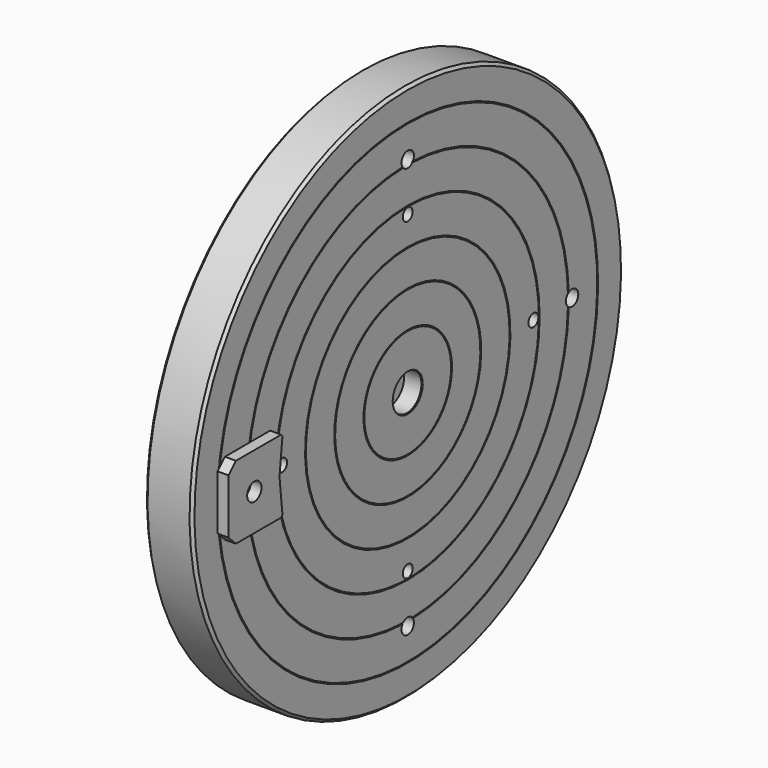
from build123d import *

# Parameters (mm, degrees)
F3_D            = 8.5
F3_DEPTH        = 20
F3_TIP          = 2.5536576309
F6_SIZE         = 1.5
F8_D            = 6.8
F10_D           = 8.5
F10_CBORE_D     = 20
F10_CBORE_DEPTH = 10
F12_D           = 8.5
F12_DEPTH       = 20
F12_TIP         = 2.5536576309
F13_R           = 4.9
F14_DEPTH       = 6
F15_SIZE        = 5
F16_SIZE        = 1


with BuildPart() as f1:
    # F0 (on Front) → F1 (revolve)
    with BuildSketch(Plane.XZ):
        Polygon((0, 80), (0, 62.5), (4, 62.5), (4, 0), (28, 0), (28, 147.5), (2, 147.5), (2, 80), align=None)
    revolve(axis=Axis((16, 0, 0), (1, 0, 0)))

    # F3
    with Locations(Plane(origin=(0, 0, 0), x_dir=(0, -1, 0), z_dir=(-1, 0, 0))):
        with Locations((0, 70), (60.6217782649, 35), (60.6217782649, -35), (0, -70), (-60.6217782649, -35), (-60.6217782649, 35)):
            Hole(F3_D / 2, depth=F3_DEPTH)
            with Locations((0, 0, -(F3_DEPTH + F3_TIP / 2))):  # 118° drill point
                Cone(0, F3_D / 2, F3_TIP, mode=Mode.SUBTRACT)

    # F4 (on Front) → F5 (revolve, cut)
    with BuildSketch(Plane.XZ):
        Polygon((28, 9.7113248654), (28, 10.2886751346), (27.5, 10), align=None)
        Polygon((28, 29.7113248654), (28, 30.2886751346), (27.5, 30), align=None)
        Polygon((28, 49.7113248654), (28, 50.2886751346), (27.5, 50), align=None)
        Polygon((28, 69.7113248654), (28, 70.2886751346), (27.5, 70), align=None)
        Polygon((28, 89.7113248654), (28, 90.2886751346), (27.5, 90), align=None)
        Polygon((28, 109.7113248654), (28, 110.2886751346), (27.5, 110), align=None)
        Polygon((28, 129.7113248654), (28, 130.2886751346), (27.5, 130), align=None)
        Polygon((28, 149.7113248654), (28, 150.2886751346), (27.5, 150), align=None)
        Polygon((28, 169.7113248654), (28, 170.2886751346), (27.5, 170), align=None)
        Polygon((28, 189.7113248654), (28, 190.2886751346), (27.5, 190), align=None)
        Polygon((28, 209.7113248654), (28, 210.2886751346), (27.5, 210), align=None)
        Polygon((28, 229.7113248654), (28, 230.2886751346), (27.5, 230), align=None)
        Polygon((28, 249.7113248654), (28, 250.2886751346), (27.5, 250), align=None)
        Polygon((28, 269.7113248654), (28, 270.2886751346), (27.5, 270), align=None)
    revolve(axis=Axis((14, 0, 0), (-1, 0, 0)), mode=Mode.SUBTRACT)

    # F6
    f6_edges = [f1.edges().sort_by_distance(p)[0] for p in [
        (28, 0, -147.5),
        (2, 0, -147.5),
    ]]
    chamfer(f6_edges, length=F6_SIZE)

    # F8 (through all)
    with Locations(Plane.YZ.offset(28)):
        with Locations((0, 86), (86, 0), (0, -86), (-86, 0)):
            Hole(F8_D / 2)

    # F10 (through all)
    with Locations(Plane.YZ.offset(28)):
        with Locations((0, 0)):
            CounterBoreHole(F10_D / 2, F10_CBORE_D / 2, F10_CBORE_DEPTH)

    # F12
    with Locations(Plane.YZ.offset(28)):
        with Locations((0, 112.5), (112.5, 0), (0, -112.5), (-112.5, 0)):
            Hole(F12_D / 2, depth=F12_DEPTH)
            with Locations((0, 0, -(F12_DEPTH + F12_TIP / 2))):  # 118° drill point
                Cone(0, F12_D / 2, F12_TIP, mode=Mode.SUBTRACT)


with BuildPart() as f14:
    # F13 (on face) → F14 (new body)
    with BuildSketch(Plane.YZ.offset(28)):
        Polygon((-93.1596355268, 20), (-130.1596355268, 20), (-130.1596355268, -20), (-93.1596355268, -20), (-95.282, 0), align=None)
        with Locations((-112.5, 0)):
            Circle(F13_R, mode=Mode.SUBTRACT)
    extrude(amount=F14_DEPTH)

    # F15
    f15_edges = [f14.edges().sort_by_distance(p)[0] for p in [
        (31, -130.159636, 20),
        (31, -130.159636, -20),
    ]]
    chamfer(f15_edges, length=F15_SIZE)

    # F16
    f16_edges = [f14.edges().sort_by_distance(p)[0] for p in [
        (31, -93.159636, 20),
        (31, -93.159636, -20),
    ]]
    chamfer(f16_edges, length=F16_SIZE)


solid = Compound([f1.part, f14.part])
